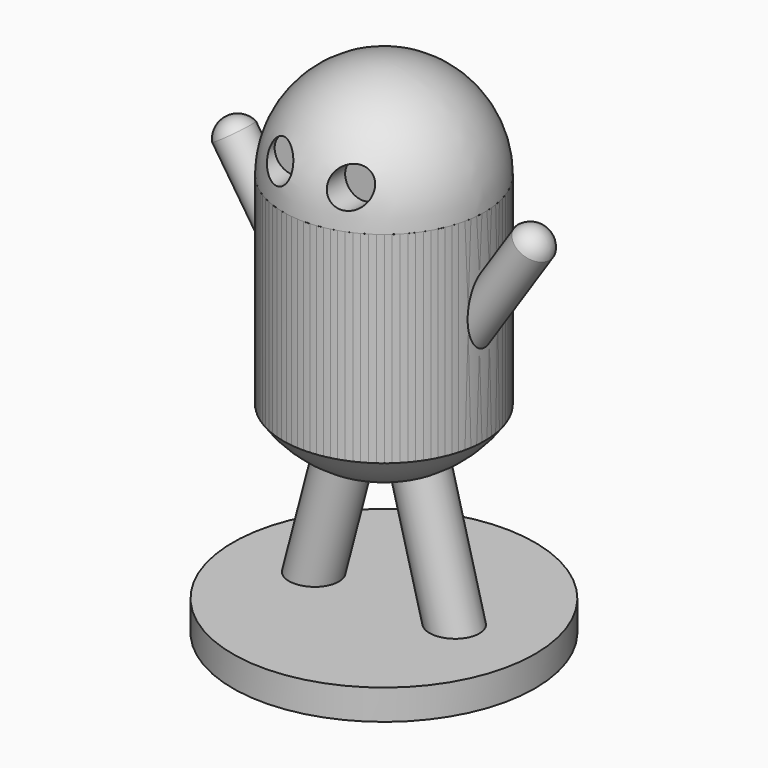
from build123d import *

# Parameters (mm, degrees)
F0_R      = 0.875
F4_R      = 0.875
F5_DEPTH  = 1.5
F9_R      = 7.5
F10_DEPTH = 1.5


with BuildPart() as f1:
    # F0 (on Front) → F1 (revolve)
    with BuildSketch(Plane.XZ):
        with BuildLine():
            Line((0, 7.5), (0, 2.5))
            Line((0, 2.5), (5, 2.5))
            ThreePointArc((5, 2.5), (3.5355339059, 6.0355339059), (0, 7.5))
        make_face()
        with Locations((1.75, 4.25)):
            Circle(F0_R, mode=Mode.SUBTRACT)
    revolve(axis=Axis((0, 0, 3.75), (0, 0, -1)))

    # F4 (on offset) → F5 (cut)
    with BuildSketch(Plane.XZ.offset(5)):
        with Locations((-1.75, 4.25)):
            Circle(F4_R)
        with Locations((1.75, 4.25)):
            Circle(F4_R)
    extrude(amount=-F5_DEPTH, mode=Mode.SUBTRACT)


with BuildPart() as f2:
    # F0 (on Front) → F2 (revolve)
    with BuildSketch(Plane.XZ):
        Polygon((5, 2.5), (0, 2.5), (0, 0), (0, -7.5), (1.25, -7.5), (2.5, -7.5), (5, -7.5), (5, -3.4158665221), (5, -1.7079332611), (5, 0), align=None)
    revolve(axis=Axis((0, 0, 3.75), (0, 0, -1)))

    # F0 (on Front) → F6 (revolve)
    with BuildSketch(Plane.XZ):
        Polygon((7.4450306957, 1.9781418576), (5, -1.7079332611), (5, -3.4158665221), (8.2317726852, 1.4562837153), align=None)
        with BuildLine():
            Line((7.8155500984, 2.5367288536), (7.4450306957, 1.9781418576))
            Line((7.4450306957, 1.9781418576), (8.2317726852, 1.4562837153))
            ThreePointArc((8.2317726852, 1.4562837153), (8.1959373098, 2.0628725678), (7.8155500984, 2.5367288536))
        make_face()
    revolve(axis=Axis((6.2225153478, 0, 0.1351042983), (0.5527653148, 0, 0.8333369707)))


with BuildPart() as f7_1:
    # F7: instance of F2
    add(f2.part.mirror(Plane.YZ))


with BuildPart() as f10:
    # F9 (on offset) → F10 (new body)
    with BuildSketch(Plane.XY.offset(-16)):
        Circle(F9_R)
    extrude(amount=-F10_DEPTH)


with BuildPart() as f11:
    # F0 (on Front) → F11 (revolve)
    with BuildSketch(Plane.XZ):
        with BuildLine():
            ThreePointArc((1.8769088058, -9.882253462), (1.2927950528, -10.0424434761), (0.6955073693, -10.1429280032))
            Line((0.6955073693, -10.1429280032), (2.5, -17))
            Line((2.5, -17), (3.75, -17))
            Line((3.75, -17), (1.8769088058, -9.882253462))
        make_face()
        with BuildLine():
            Line((1.25, -7.5), (0, -7.5))
            Line((0, -7.5), (0.6955073693, -10.1429280032))
            ThreePointArc((0.6955073693, -10.1429280032), (1.2927950528, -10.0424434761), (1.8769088058, -9.882253462))
            Line((1.8769088058, -9.882253462), (1.25, -7.5))
        make_face()
    revolve(axis=Axis((2.5, 0, -12.25), (-0.2544932993, 0, 0.9670745373)))


with BuildPart() as f12:
    # F0 (on Front) → F12 (revolve)
    with BuildSketch(Plane.XZ):
        with BuildLine():
            Line((-2.5, -17), (-0.6955073693, -10.1429280032))
            ThreePointArc((-0.6955073693, -10.1429280032), (-1.2927950528, -10.0424434761), (-1.8769088058, -9.882253462))
            Line((-1.8769088058, -9.882253462), (-3.75, -17))
            Line((-3.75, -17), (-2.5, -17))
        make_face()
        with BuildLine():
            Line((-0.6955073693, -10.1429280032), (0, -7.5))
            Line((0, -7.5), (-1.25, -7.5))
            Line((-1.25, -7.5), (-1.8769088058, -9.882253462))
            ThreePointArc((-1.8769088058, -9.882253462), (-1.2927950528, -10.0424434761), (-0.6955073693, -10.1429280032))
        make_face()
    revolve(axis=Axis((-2.5, 0, -12.25), (0.2544932993, 0, 0.9670745373)))


with BuildPart() as f13:
    # F0 (on Front) → F13 (revolve)
    with BuildSketch(Plane.XZ):
        with BuildLine():
            Line((0.6955073693, -10.1429280032), (0, -7.5))
            Line((0, -7.5), (0, -9.4098300563))
            Line((0, -9.4098300563), (0, -10.1833752096))
            ThreePointArc((0, -10.1833752096), (0.3483412397, -10.1732548729), (0.6955073693, -10.1429280032))
        make_face()
        with BuildLine():
            Line((1.25, -7.5), (0, -7.5))
            Line((0, -7.5), (0.6955073693, -10.1429280032))
            ThreePointArc((0.6955073693, -10.1429280032), (1.2927950528, -10.0424434761), (1.8769088058, -9.882253462))
            Line((1.8769088058, -9.882253462), (1.25, -7.5))
        make_face()
        with BuildLine():
            Line((-1.8769088058, -9.882253462), (-1.25, -7.5))
            Line((-1.25, -7.5), (-5, -7.5))
            ThreePointArc((-5, -7.5), (-3.6389217593, -8.9539358088), (-1.8769088058, -9.882253462))
        make_face()
        with BuildLine():
            Line((2.5, -7.5), (1.25, -7.5))
            Line((1.25, -7.5), (1.8769088058, -9.882253462))
            ThreePointArc((1.8769088058, -9.882253462), (3.6389217593, -8.9539358088), (5, -7.5))
            Line((5, -7.5), (2.5, -7.5))
        make_face()
    revolve(axis=Axis((0, 0, -8.8416876048), (0, 0, -1)))


solid = Compound([f1.part, f2.part, f7_1.part, f10.part, f11.part, f12.part, f13.part])
